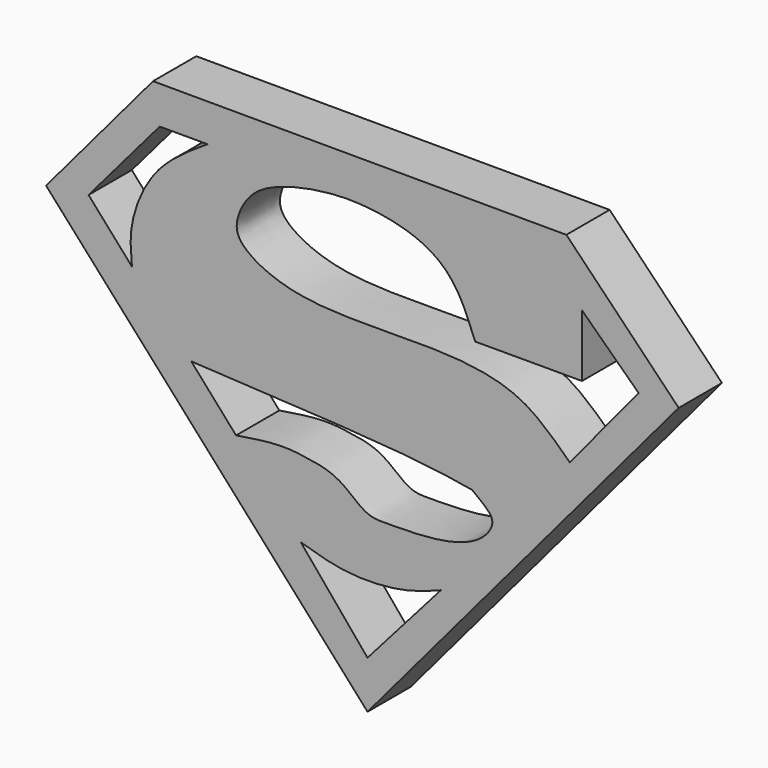
from build123d import *

# Parameters (mm, degrees)
F1_DEPTH = 5


with BuildPart() as f1:
    # F0 (on Front) → F1 (new body)
    with BuildSketch(Plane.XZ):
        Polygon((6.8467608653, 29.1649848223), (-31.379327178, 29.241707176), (-41.2686094642, 17.5228919834), (-11.5442769602, -15.64797014), (17.2308642175, 18.4506177902), align=None)
        with BuildLine():
            Line((-23.6961469054, 2.9009203427), (-27.847610414, 7.5846225955))
            add(Edge.make_bspline(
                [(-27.847610414, 7.5846225955), (-19.8370461585, 7.1792182284), (-7.743850984, 6.5671971549), (-3.3557602446, 5.8157885618), (-1.8743523397, 5.562114995)],
                knots=[0, 0, 0, 0, 0.6624026273, 1, 1, 1, 1], degree=3))
            add(Edge.make_bspline(
                [(-1.8743523397, 5.562114995), (-1.4179422708, 5.2205821712), (-0.585004998, 4.5972930761), (0.3331977784, 3.5560373112), (-1.010582746, 1.5006672697), (-4.7068912366, 0.3001401954), (-9.3254664772, 0.2750656567), (-11.5190753977, 0.2264516302), (-13.1447218731, 1.6614626896), (-14.7675912552, 2.7897659842), (-17.1739824037, 3.2404166307), (-19.8261847392, 3.523178168), (-22.3243012801, 3.1215017434), (-23.6961469054, 2.9009203427)],
                knots=[0, 0, 0, 0, 0.0742843887, 0.1355672023, 0.2162485732, 0.3309490429, 0.4559254615, 0.5393908146, 0.6210669212, 0.7022428758, 0.790900937, 0.8851728372, 1, 1, 1, 1], degree=3))
        make_face(mode=Mode.SUBTRACT)
        with BuildLine():
            Line((-11.5442769602, -11.2505741417), (-17.7106130868, -3.8509704173))
            add(Edge.make_bspline(
                [(-17.7106130868, -3.8509704173), (-16.3226608848, -4.2718337351), (-13.4481313377, -5.1434660871), (-8.2276905085, -4.8931100883), (-5.8513779321, -3.9673311063), (-4.7613061033, -3.5426539835)],
                knots=[0, 0, 0, 0, 0.3357095554, 0.695273969, 1, 1, 1, 1], degree=3))
            Line((-4.7613061033, -3.5426539835), (-11.5442769602, -11.2505741417))
        make_face(mode=Mode.SUBTRACT)
        with BuildLine():
            Line((-37.3401194811, 18.0395282805), (-30.7626947761, 25.7474500686))
            Line((-30.7626947761, 25.7474500686), (-26.3434872031, 25.7474500686))
            add(Edge.make_bspline(
                [(-33.3320014179, 13.5175473988), (-33.4352493357, 14.5816524239), (-33.6697363916, 16.998348661), (-31.4985236243, 22.4095155368), (-28.0944284632, 24.6136991466), (-26.3434872031, 25.7474500686)],
                knots=[0, 0, 0, 0, 0.2764414704, 0.6278281236, 1, 1, 1, 1], degree=3))
            Line((-33.3320014179, 13.5175473988), (-37.3401194811, 18.0395282805))
        make_face(mode=Mode.SUBTRACT)
        with BuildLine():
            Line((8.2907760516, 17.7312102169), (8.2907760516, 23.4864596277))
            Line((8.2907760516, 23.4864596277), (13.5321617126, 18.4506177902))
            Line((13.5321617126, 18.4506177902), (7.1602808312, 10.7426950708))
            add(Edge.make_bspline(
                [(-1.5753639163, 17.7312102169), (-2.1681666347, 19.2227640195), (-3.3125827283, 22.1022349186), (-6.6744835027, 24.6564570993), (-12.3505834457, 25.7354953948), (-17.3440689805, 25.2648643198), (-21.9570699991, 23.8168081138), (-23.5944944017, 21.0759037774), (-23.8438395799, 18.743270129), (-19.7163395181, 16.3201047984), (-13.6718770191, 15.7522211208), (-6.8063195481, 15.9645316546), (-1.6258813787, 15.7606132749), (3.1922483306, 14.5681097618), (5.8065686961, 12.0477524987), (7.1602808312, 10.7426950708)],
                knots=[0, 0, 0, 0, 0.0767260342, 0.1481209611, 0.2327425226, 0.3140883717, 0.3908631304, 0.4521063897, 0.5012736199, 0.5740049671, 0.6637506815, 0.7576500248, 0.8389855697, 0.9166256779, 1, 1, 1, 1], degree=3))
            Line((-1.5753639163, 17.7312102169), (8.2907760516, 17.7312102169))
        make_face(mode=Mode.SUBTRACT)
    extrude(amount=F1_DEPTH)


solid = f1.part
